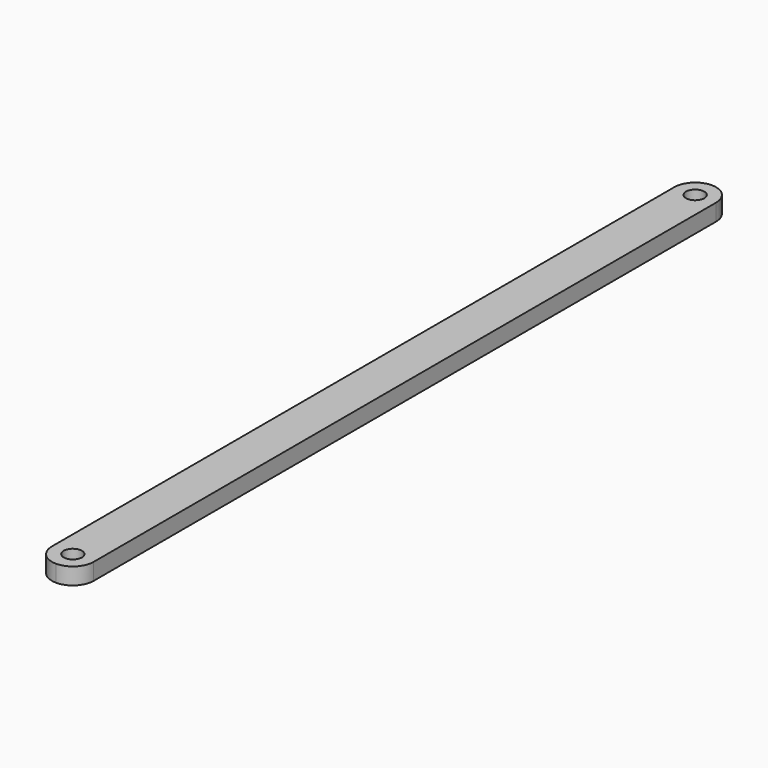
from build123d import *

# Parameters (mm, degrees)
F0_W     = 7.9375
F0_H     = 155.575
F1_DEPTH = 3.175
F2_R     = 1.7272
F3_DEPTH = 3.175
F4_R     = 3.96874


# Not quite as in the source:
# - a fillet or chamfer is up to 0.001 mm smaller than in the source, because OpenCascade refuses the exact size


with BuildPart() as f1:
    # F0 (on Top) → F1 (new body)
    with BuildSketch(Plane.XY):
        Rectangle(F0_W, F0_H)
    extrude(amount=F1_DEPTH)

    # F2 (on face) → F3 (cut, through all)
    with BuildSketch(Plane.XY.offset(3.175)):
        with Locations((0, 73.81875)):
            Circle(F2_R)
        with Locations((0, -73.81875)):
            Circle(F2_R)
    extrude(amount=-F3_DEPTH, mode=Mode.SUBTRACT)

    # F4 (radius 3.96875 in the source; OpenCascade refuses exactly that, so slightly less here)
    f4_edges = [f1.edges().sort_by_distance(p)[0] for p in [
        (-3.96875, -77.7875, 1.5875),
        (3.96875, -77.7875, 1.5875),
        (3.96875, 77.7875, 1.5875),
        (-3.96875, 77.7875, 1.5875),
    ]]
    fillet(f4_edges, radius=F4_R)


solid = f1.part
